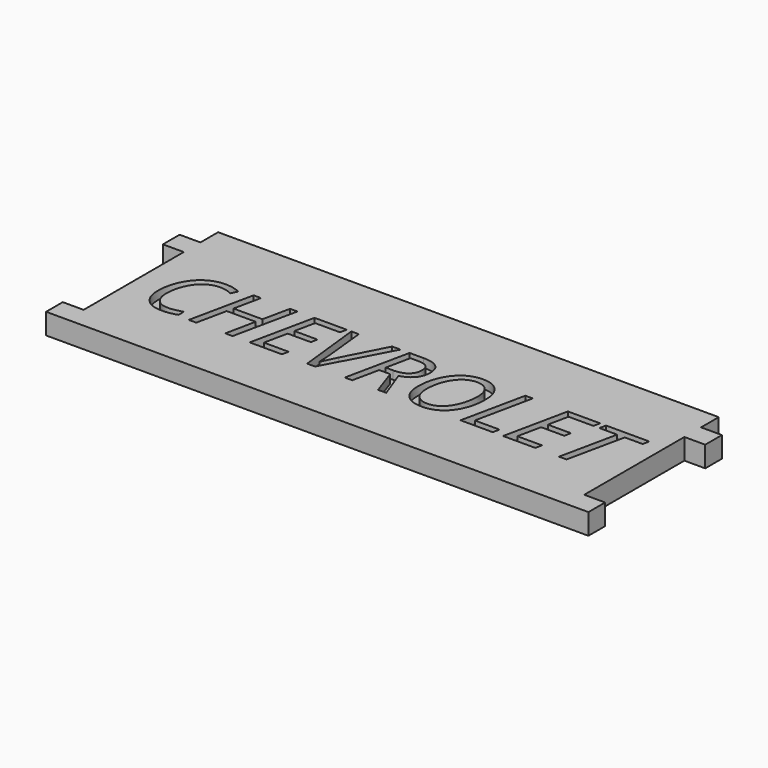
from build123d import *

# Parameters (mm, degrees)
F1_DEPTH     = 5
F2_TEXT_SIZE = 21.522297498
F3_DEPTH     = 2


# Not quite as in the source:
# - Text() gives the source's letters only with a copy of the font that has no kerning and outlines rounded to 1/6400 em; it was checked with that copy


with BuildPart() as f1:
    # F0 (on Top) → F1 (new body)
    with BuildSketch(Plane.XY):
        Polygon((60, 17.35), (60, 22.65), (-60, 22.65), (-60, 17.35), (-65, 17.35), (-65, 12.35), (-60, 12.35), (-60, -17.65), (-65, -17.65), (-65, -22.65), (-60, -22.65), (60, -22.65), (65, -22.65), (65, -17.65), (60, -17.65), (60, 12.35), (65, 12.35), (65, 17.35), align=None)
    extrude(amount=F1_DEPTH)

    # F2 (on face) → F3 (cut)
    with BuildSketch(Plane.XY.offset(5)):
        with Locations((-55.5789098144, -8.5406622384)):
            Text('CHEVROLET', F2_TEXT_SIZE, font='Open Sans', font_style=FontStyle.ITALIC, text_align=(TextAlign.LEFT, TextAlign.BOTTOM))
    extrude(amount=-F3_DEPTH, mode=Mode.SUBTRACT)


solid = f1.part
